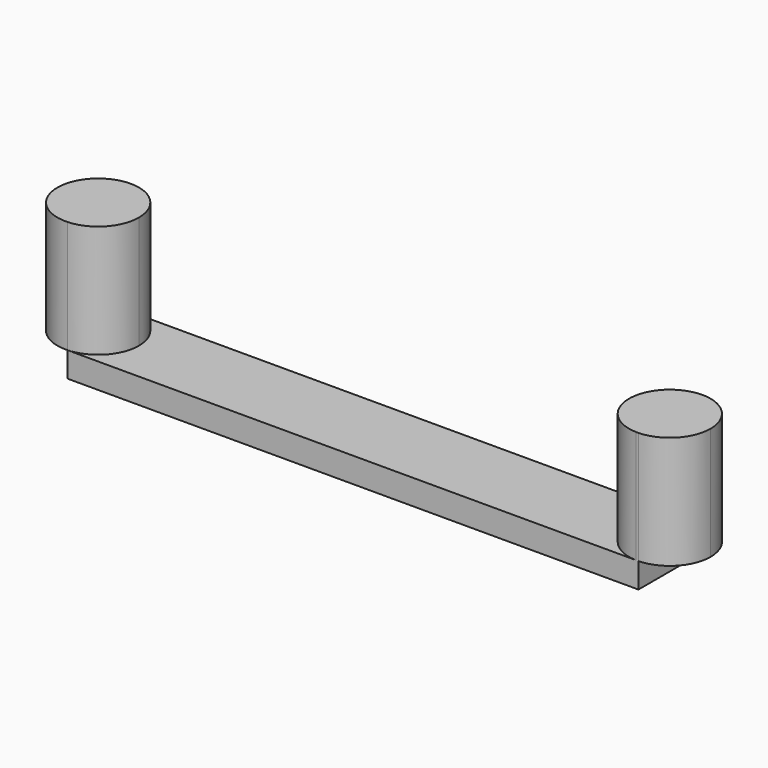
from build123d import *

# Parameters (mm, degrees)
F1_DEPTH = 114.3
F2_DEPTH = 25.4


with BuildPart() as f1:
    # F0 (on Top) → F1 (new body)
    with BuildSketch(Plane.XY):
        with BuildLine():
            ThreePointArc((400.6691527557, 0), (387.8651300869, 29.8835920667), (357.3969989189, 41.2266540184))
            Line((357.3969989189, 41.2266540184), (360.6180139352, 41.2266540184))
            Line((360.6180139352, 41.2266540184), (360.6180139352, -41.2568514166))
            ThreePointArc((360.6180139352, -41.2568514166), (389.0095245682, -28.7498761286), (400.6691527557, 0))
        make_face()
        with BuildLine():
            Line((360.6180139352, 41.2266540184), (357.3969989189, 41.2266540184))
            ThreePointArc((357.3969989189, 41.2266540184), (318.1209665249, -0.3869410216), (358.1702915763, -41.2568514166))
            Line((358.1702915763, -41.2568514166), (360.6180139352, -41.2568514166))
            Line((360.6180139352, -41.2568514166), (360.6180139352, 41.2266540184))
        make_face()
    extrude(amount=F1_DEPTH)



with BuildPart() as f1b:
    # F0 (on Top) → F1, piece 2 (new body)
    with BuildSketch(Plane.XY):
        with BuildLine():
            Line((-217.7286934074, -41.2266540184), (-217.7286934074, 41.2266540184))
            ThreePointArc((-217.7286934074, 41.2266540184), (-261.0008472443, 0), (-217.7286934074, -41.2266540184))
        make_face()
        with BuildLine():
            ThreePointArc((-217.7286934074, -41.2266540184), (-189.8422551776, -28.4709773312), (-178.4508472443, 0))
            ThreePointArc((-178.4508472443, 0), (-189.8422551776, 28.4709773312), (-217.7286934074, 41.2266540184))
            Line((-217.7286934074, 41.2266540184), (-217.7286934074, -41.2266540184))
        make_face()
    extrude(amount=F1_DEPTH)


with BuildPart() as f1_1:
    add(f1.part)

    add(f1b.part)  # F2 merges F1b
    # F0 (on Top) → F2 (join)
    with BuildSketch(Plane.XY):
        with BuildLine():
            ThreePointArc((-217.7286934074, -41.2266540184), (-189.8422551776, -28.4709773312), (-178.4508472443, 0))
            ThreePointArc((-178.4508472443, 0), (-189.8422551776, 28.4709773312), (-217.7286934074, 41.2266540184))
            Line((-217.7286934074, 41.2266540184), (-217.7286934074, -41.2266540184))
        make_face()
        with BuildLine():
            ThreePointArc((-217.7286934074, 41.2266540184), (-189.8422551776, 28.4709773312), (-178.4508472443, 0))
            ThreePointArc((-178.4508472443, 0), (-189.8422551776, -28.4709773312), (-217.7286934074, -41.2266540184))
            Line((-217.7286934074, -41.2266540184), (-217.7286934074, -41.2568514166))
            Line((-217.7286934074, -41.2568514166), (358.1702915763, -41.2568514166))
            ThreePointArc((358.1702915763, -41.2568514166), (318.1209665249, -0.3869410216), (357.3969989189, 41.2266540184))
            Line((357.3969989189, 41.2266540184), (-217.7286934074, 41.2266540184))
        make_face()
        with BuildLine():
            Line((360.6180139352, 41.2266540184), (357.3969989189, 41.2266540184))
            ThreePointArc((357.3969989189, 41.2266540184), (318.1209665249, -0.3869410216), (358.1702915763, -41.2568514166))
            Line((358.1702915763, -41.2568514166), (360.6180139352, -41.2568514166))
            Line((360.6180139352, -41.2568514166), (360.6180139352, 41.2266540184))
        make_face()
    extrude(amount=-F2_DEPTH)


solid = f1_1.part
